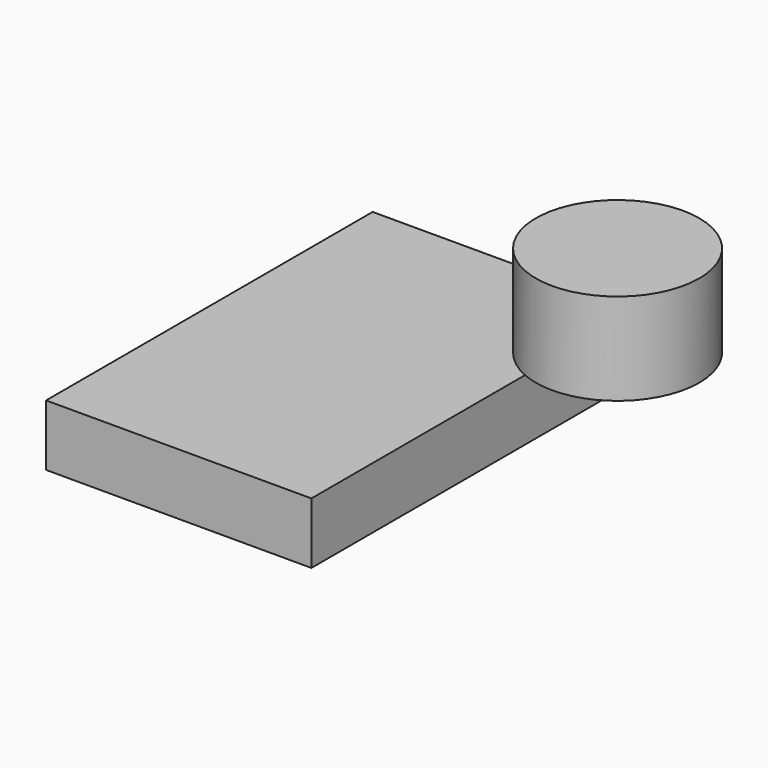
from build123d import *

# Parameters (mm, degrees)
F1_DEPTH = 63.5


# Not quite as in the source:
# - a feature of the source that left no trace in its solid (it failed there, or was rolled back) is left out


with BuildPart() as f1:
    # F0 (on Front) → F1 (new body, symmetric)
    with BuildSketch(Plane.XZ):
        Polygon((22.225, 9.525), (-41.275, 9.525), (-41.275, -9.525), (41.275, -9.525), (41.275, 9.525), align=None)
    extrude(amount=F1_DEPTH, both=True)


with BuildPart() as f2:
    # F0 (on Front) → F2 (revolve)
    with BuildSketch(Plane.XZ):
        Polygon((85.725, 66.675), (85.725, 61.9252), (85.725, 42.8752), (85.725, 38.1), (111.125, 38.1), (111.125, 66.675), align=None)
    revolve(axis=Axis((85.725, 0, 52.3875), (0, 0, 1)))


solid = Compound([f1.part, f2.part])
